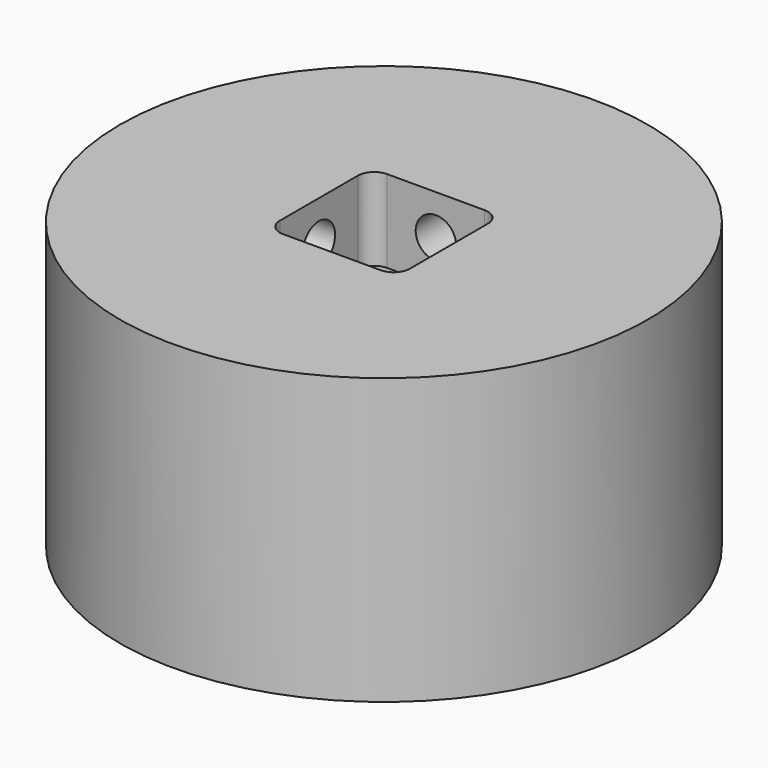
from build123d import *

# Parameters (mm, degrees)
F3_DEPTH        = 25
F4_R            = 2.5
F5_DEPTH        = 24.571
F5_COPIES_COUNT = 2
F5_COPIES_ANGLE = 270


# Not quite as in the source:
# - a pattern or mirror of a feature is missing from the dataset's text; its kind, count and spacing are read off the source's solid


with BuildPart() as f1:
    # F0 (on Front) → F1 (revolve)
    with BuildSketch(Plane.XZ):
        Polygon((0, -10.2), (0, 0), (-32.6, 0), (-32.6, -35.2), (-30.25, -35.2), (-27.25, -32.2), (-29.6, -32.2), (-29.6, -10.2), align=None)
    revolve(axis=Axis((0, 0, -5.1), (0, 0, 1)))

    # F2 (on face) → F3 (cut)
    with BuildSketch(Plane.XY):
        with BuildLine():
            ThreePointArc((8.03, 6.03), (7.4442135624, 7.4442135624), (6.03, 8.03))
            Line((6.03, 8.03), (-6.03, 8.03))
            ThreePointArc((-6.03, 8.03), (-7.4442135624, 7.4442135624), (-8.03, 6.03))
            Line((-8.03, 6.03), (-8.03, -6.03))
            ThreePointArc((-8.03, -6.03), (-7.4442135624, -7.4442135624), (-6.03, -8.03))
            Line((-6.03, -8.03), (6.03, -8.03))
            ThreePointArc((6.03, -8.03), (7.4442135624, -7.4442135624), (8.03, -6.03))
            Line((8.03, -6.03), (8.03, 6.03))
        make_face()
    extrude(amount=-F3_DEPTH, mode=Mode.SUBTRACT)

    # F4 (on face) → F5 (cut, through all)
    with BuildSketch(Plane.YZ.offset(-8.03)):
        with Locations((0, -5)):
            Circle(F4_R)
    f5 = extrude(amount=-F5_DEPTH, mode=Mode.SUBTRACT)

    # F5_copies: F5 ×2 about axis
    f5_copies_axis = Axis((0, 0, 0), (0, 0, 1))
    for i in range(1, F5_COPIES_COUNT):
        add(f5.rotate(f5_copies_axis, i * F5_COPIES_ANGLE / (F5_COPIES_COUNT - 1)), mode=Mode.SUBTRACT)


solid = f1.part
